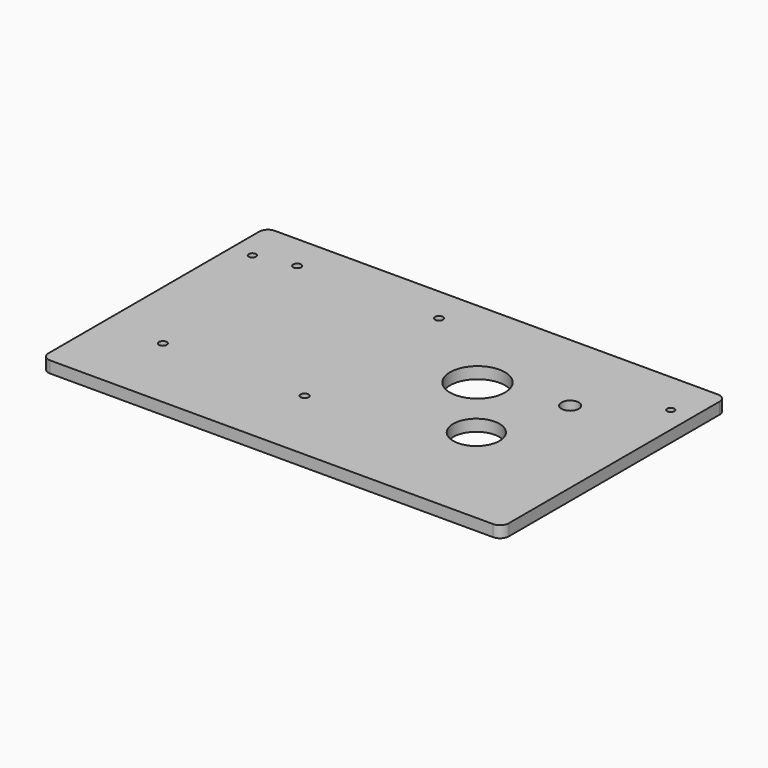
from build123d import *

# Parameters (mm, degrees)
F0_R     = 1.375
F0_R_2   = 1.25
F0_R_3   = 8
F0_R_4   = 9.5
F0_R_5   = 3
F1_DEPTH = 4
F2_R     = 3


with BuildPart() as f1:
    # F0 (on Top) → F1 (new body)
    with BuildSketch(Plane.XY):
        with BuildLine():
            Line((-4.7679491924, -48.5), (79.5, -48.5))
            Line((79.5, -48.5), (79.5, 48.5))
            Line((79.5, 48.5), (-79.5, 48.5))
            Line((-79.5, 48.5), (-79.5, -48.5))
            Line((-79.5, -48.5), (-64.2320508076, -48.5))
            ThreePointArc((-64.2320508076, -48.5), (-62.5, -47.5), (-60.7679491924, -48.5))
            Line((-60.7679491924, -48.5), (-8.2320508076, -48.5))
            ThreePointArc((-8.2320508076, -48.5), (-6.5, -47.5), (-4.7679491924, -48.5))
        make_face()
        with Locations((-59, -21.75)):
            Circle(F0_R, mode=Mode.SUBTRACT)
        with Locations((-10, -21.75)):
            Circle(F0_R, mode=Mode.SUBTRACT)
        with Locations((-72.275, 33.5)):
            Circle(F0_R_2, mode=Mode.SUBTRACT)
        with Locations((-59, 36.25)):
            Circle(F0_R, mode=Mode.SUBTRACT)
        with Locations((-10, 36.25)):
            Circle(F0_R, mode=Mode.SUBTRACT)
        with Locations((39.5, -9.5)):
            Circle(F0_R_3, mode=Mode.SUBTRACT)
        with Locations((21.5, 13.5)):
            Circle(F0_R_4, mode=Mode.SUBTRACT)
        with Locations((49.5, 18.5)):
            Circle(F0_R_5, mode=Mode.SUBTRACT)
        with Locations((72.275, 33.5)):
            Circle(F0_R_2, mode=Mode.SUBTRACT)
        with BuildLine():
            Line((-8.2320508076, -48.5), (-4.7679491924, -48.5))
            ThreePointArc((-4.7679491924, -48.5), (-6.5, -47.5), (-8.2320508076, -48.5))
        make_face()
        with BuildLine():
            Line((-64.2320508076, -48.5), (-60.7679491924, -48.5))
            ThreePointArc((-60.7679491924, -48.5), (-62.5, -47.5), (-64.2320508076, -48.5))
        make_face()
    extrude(amount=F1_DEPTH)

    # F2
    f2_edges = [f1.edges().sort_by_distance(p)[0] for p in [
        (-79.5, 48.5, 2),
        (79.5, 48.5, 2),
        (79.5, -48.5, 2),
        (-79.5, -48.5, 2),
    ]]
    fillet(f2_edges, radius=F2_R)


solid = f1.part
